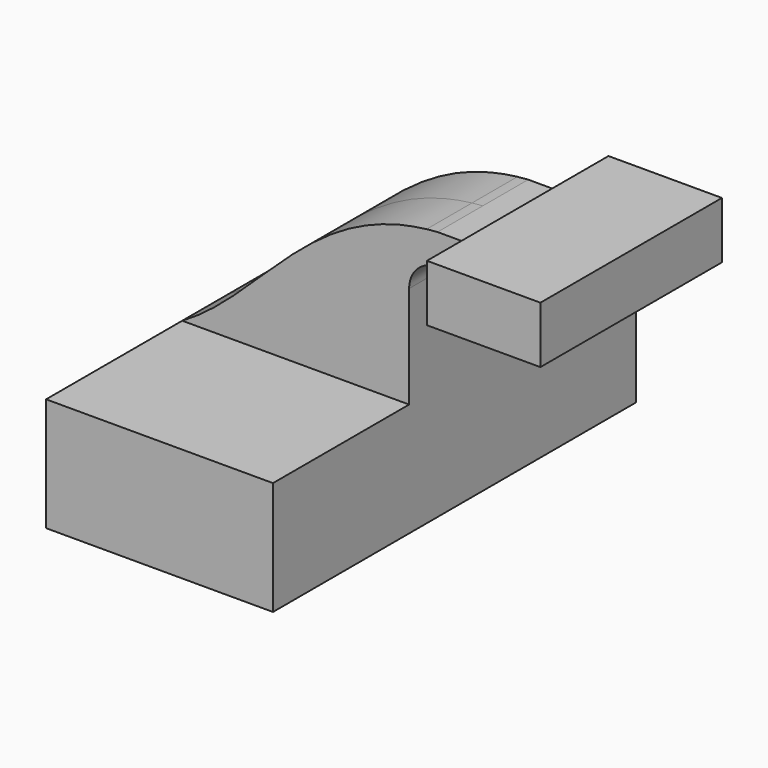
from build123d import *

# Parameters (mm, degrees)
F0_W     = 50.8
F0_H     = 25.4
F1_DEPTH = 50.8
F0_W_2   = 15.5147364107
F0_H_2   = 3.81
F0_H_3   = 2.0320005715
F0_H_4   = 6.8579994285
F2_DEPTH = 25.4
F3_DEPTH = 12.7


with BuildPart() as f1:
    # F0 (on Front) → F1 (new body, symmetric)
    with BuildSketch(Plane.XZ):
        with Locations((0, -0.3042038961)):
            Rectangle(F0_W, F0_H)
    extrude(amount=F1_DEPTH, both=True)

    # F0 (on Front) → F3 (join, symmetric)
    with BuildSketch(Plane.XZ):
        with BuildLine():
            Line((39.5527683854, 41.6057961039), (39.5527683854, 48.4637955324))
            Line((39.5527683854, 48.4637955324), (31.75, 48.4637955324))
            add(Edge.make_bspline(
                [(29.3220054539, 48.2387114694), (30.116500968, 48.3313826288), (30.9256164541, 48.4066923242), (31.75, 48.4637955324)],
                knots=[65.6114978001, 65.6114978001, 65.6114978001, 65.6114978001, 67.5797534974, 67.5797534974, 67.5797534974, 67.5797534974], degree=3))
            add(Edge.make_bspline(
                [(-25.4, 12.3957961039), (-7.4008771224, 22.7680893729), (2.8376209581, 45.1495327735), (29.3220054539, 48.2387114694)],
                knots=[0, 0, 0, 0, 65.6114978001, 65.6114978001, 65.6114978001, 65.6114978001], degree=3))
            Line((-25.4, 12.3957961039), (25.4, 12.3957961039))
            Line((25.4, 12.3957961039), (25.4, 35.2557961039))
            ThreePointArc((25.4, 35.2557961039), (27.2598719395, 39.7459241644), (31.75, 41.6057961039))
            Line((31.75, 41.6057961039), (39.5527683854, 41.6057961039))
        make_face()
    extrude(amount=F3_DEPTH, both=True)


with BuildPart() as f2:
    # F0 (on Front) → F2 (new body, symmetric)
    with BuildSketch(Plane.XZ):
        Polygon((64.9527683854, 50.4957961039), (55.0675047961, 50.4957961039), (55.0675047961, 48.4637955324), (55.0675047961, 41.6057961039), (55.0675047961, 37.7957961039), (64.9527683854, 37.7957961039), align=None)
        with Locations((47.3101365908, 39.7007961039)):
            Rectangle(F0_W_2, F0_H_2)
        with Locations((47.3101365908, 49.4797958182)):
            Rectangle(F0_W_2, F0_H_3)
        with Locations((47.3101365908, 45.0347958182)):
            Rectangle(F0_W_2, F0_H_4)
    extrude(amount=F2_DEPTH, both=True)


solid = Compound([f1.part, f2.part])
